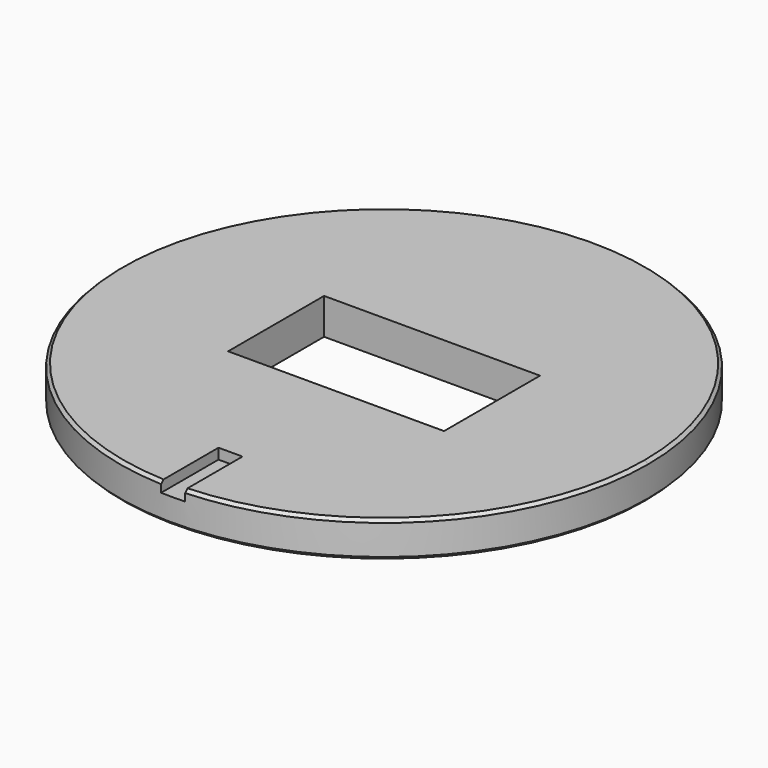
from build123d import *

# Parameters (mm, degrees)
F2_R     = 139.7
F2_R_2   = 2.9765625
F3_DEPTH = 19.05
F4_SIZE  = 1.5875
F6_W     = 12.7
F6_H     = 5.55625
F7_DEPTH = 38.1
F8_W     = 114.3
F8_H     = 63.5
F8_R     = 2.9765625
F9_DEPTH = 19.051


# Not quite as in the source:
# - a variable given as a bare number and used for a length is read in inches; the dataset says mm whatever the document's units were


with BuildPart() as f3:
    # F2 (on Top) → F3 (new body)
    with BuildSketch(Plane.XY):
        Circle(F2_R)
        Circle(F2_R_2, mode=Mode.SUBTRACT)
    extrude(amount=F3_DEPTH)

    # F4
    f4_edges = [f3.edges().sort_by_distance(p)[0] for p in [
        (-139.7, 0, 19.05),
        (-139.7, 0, 0),
    ]]
    chamfer(f4_edges, length=F4_SIZE)

    # F6 (on offset) → F7 (cut)
    with BuildSketch(Plane.XZ.offset(139.7)):
        with Locations((0, 16.271875)):
            Rectangle(F6_W, F6_H)
    extrude(amount=-F7_DEPTH, mode=Mode.SUBTRACT)

    # F8 (on face) → F9 (cut, through all)
    with BuildSketch(Plane.XY.offset(19.05)):
        Rectangle(F8_W, F8_H)
        Circle(F8_R, mode=Mode.SUBTRACT)
    extrude(amount=-F9_DEPTH, mode=Mode.SUBTRACT)


solid = f3.part
